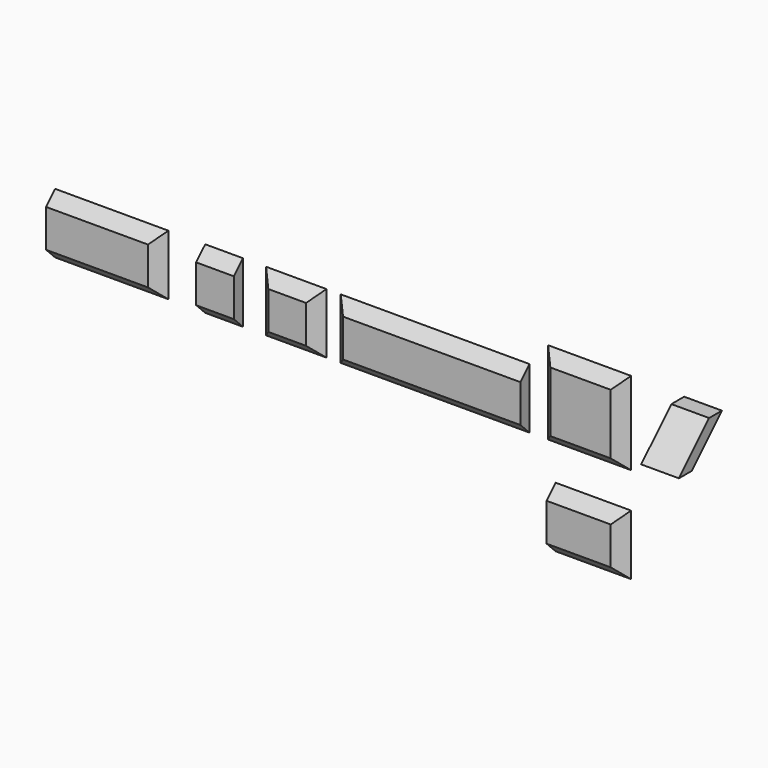
from build123d import *

# Parameters (mm, degrees)
F0_W       = 110
F0_H       = 110
F1_DEPTH   = 15
F2_W       = 250
F2_H       = 80
F3_DEPTH   = 15
F4_W       = 80
F4_H       = 80
F5_DEPTH   = 15
F6_W       = 50
F6_H       = 80
F7_DEPTH   = 15
F8_W       = 150
F8_H       = 80
F9_DEPTH   = 15
F11_DEPTH  = 50
F12_W      = 100
F12_H      = 80
F13_DEPTH  = 15
F14_SIZE   = 14.99999
F14_2_SIZE = 14.99999
F14_3_SIZE = 14.99999
F14_4_SIZE = 14.99999
F14_5_SIZE = 14.99999
F14_6_SIZE = 14.99999


# Not quite as in the source:
# - a fillet or chamfer is up to 0.001 mm smaller than in the source, because OpenCascade refuses the exact size


with BuildPart() as f1:
    # F0 (on Front) → F1 (new body)
    with BuildSketch(Plane.XZ):
        with Locations((-55, 55)):
            Rectangle(F0_W, F0_H)
    extrude(amount=F1_DEPTH)

    # F14#2 (size 15 in the source; OpenCascade refuses exactly that, so slightly less here)
    f14_2_edges = [f1.edges().sort_by_distance(p)[0] for p in [
        (-55, -15, 0),
        (0, -15, 55),
        (-55, -15, 110),
        (-110, -15, 55),
    ]]
    chamfer(f14_2_edges, length=F14_2_SIZE)


with BuildPart() as f3:
    # F2 (on Front) → F3 (new body)
    with BuildSketch(Plane.XZ):
        with Locations((-259.6421393369, 40)):
            Rectangle(F2_W, F2_H)
    extrude(amount=F3_DEPTH)

    # F14#3 (size 15 in the source; OpenCascade refuses exactly that, so slightly less here)
    f14_3_edges = [f3.edges().sort_by_distance(p)[0] for p in [
        (-259.642139, -15, 80),
        (-384.642139, -15, 40),
        (-259.642139, -15, 0),
    ]]
    chamfer(f14_3_edges, length=F14_3_SIZE)


with BuildPart() as f5:
    # F4 (on Front) → F5 (new body)
    with BuildSketch(Plane.XZ):
        with Locations((-443.5716368201, 40)):
            Rectangle(F4_W, F4_H)
    extrude(amount=F5_DEPTH)

    # F14 (size 15 in the source; OpenCascade refuses exactly that, so slightly less here)
    f14_edges = [f5.edges().sort_by_distance(p)[0] for p in [
        (-443.571637, -15, 0),
        (-403.571637, -15, 40),
        (-443.571637, -15, 80),
        (-483.571637, -15, 40),
    ]]
    chamfer(f14_edges, length=F14_SIZE)


with BuildPart() as f7:
    # F6 (on Front) → F7 (new body)
    with BuildSketch(Plane.XZ):
        with Locations((-539.1425021022, 40)):
            Rectangle(F6_W, F6_H)
    extrude(amount=F7_DEPTH)

    # F14#4 (size 15 in the source; OpenCascade refuses exactly that, so slightly less here)
    f14_4_edges = [f7.edges().sort_by_distance(p)[0] for p in [
        (-539.142502, -15, 80),
        (-539.142502, -15, 0),
    ]]
    chamfer(f14_4_edges, length=F14_4_SIZE)


with BuildPart() as f9:
    # F8 (on Front) → F9 (new body)
    with BuildSketch(Plane.XZ):
        with Locations((-687.9779948193, 40)):
            Rectangle(F8_W, F8_H)
    extrude(amount=F9_DEPTH)

    # F14#5 (size 15 in the source; OpenCascade refuses exactly that, so slightly less here)
    f14_5_edges = [f9.edges().sort_by_distance(p)[0] for p in [
        (-687.977995, -15, 0),
        (-687.977995, -15, 80),
        (-612.977995, -15, 40),
    ]]
    chamfer(f14_5_edges, length=F14_5_SIZE)


with BuildPart() as f11:
    # F10 (on Right) → F11 (new body)
    with BuildSketch(Plane.YZ):
        Polygon((66.6554310362, 50), (16.6554310362, 0), (37.8686344718, 0), (87.8686344718, 50), align=None)
    extrude(amount=F11_DEPTH)


with BuildPart() as f13:
    # F12 (on Front) → F13 (new body)
    with BuildSketch(Plane.XZ):
        with Locations((-50, -87.0886105629)):
            Rectangle(F12_W, F12_H)
    extrude(amount=F13_DEPTH)

    # F14#6 (size 15 in the source; OpenCascade refuses exactly that, so slightly less here)
    f14_6_edges = [f13.edges().sort_by_distance(p)[0] for p in [
        (0, -15, -87.088611),
        (-50, -15, -47.088611),
        (-50, -15, -127.088611),
    ]]
    chamfer(f14_6_edges, length=F14_6_SIZE)


solid = Compound([f1.part, f3.part, f5.part, f7.part, f9.part, f11.part, f13.part])
